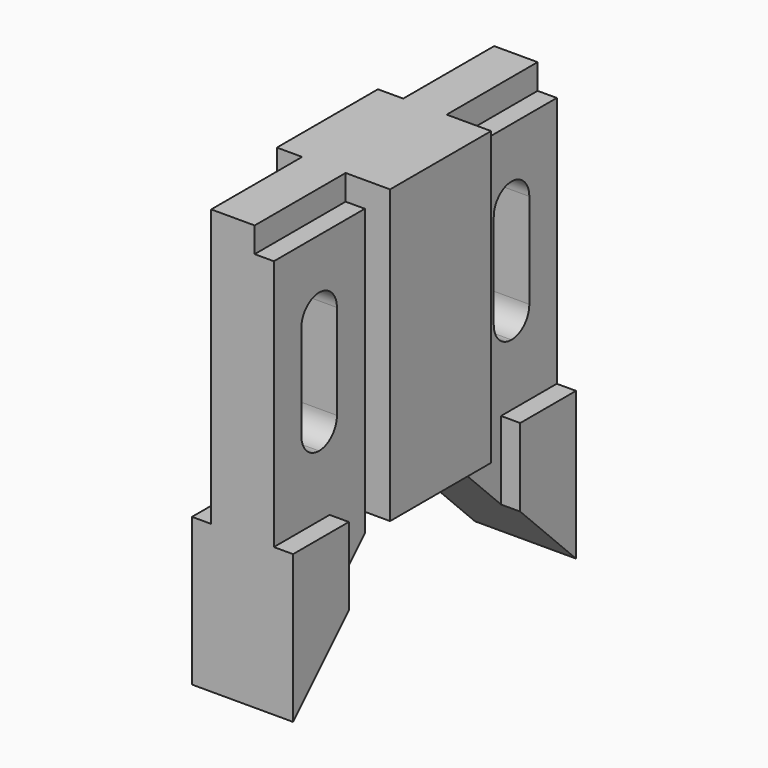
from build123d import *

# Parameters (mm, degrees)
F0_W      = 28.448
F0_H      = 73.406
F1_DEPTH  = 15.875
F2_W      = 28.575
F2_H      = 6.35
F3_DEPTH  = 7.874
F5_W      = 28.575
F5_H      = 6.35
F6_DEPTH  = 4.826
F8_DEPTH  = 12.7
F12_DEPTH = 40.132


with BuildPart() as f1:
    # F0 (on Front) → F1 (new body, symmetric)
    with BuildSketch(Plane.XZ):
        Rectangle(F0_W, F0_H)
    extrude(amount=F1_DEPTH, both=True)

    # F2 (on Right) → F3 (join, symmetric)
    with BuildSketch(Plane.YZ):
        Polygon((-15.875, -36.703), (-15.875, 30.353), (-44.45, 30.353), (-44.45, -32.893), (-26.924, -32.893), (-26.924, -52.4899314183), (-15.875, -41.4409314183), align=None)
        with Locations((-30.1625, 33.528)):
            Rectangle(F2_W, F2_H)
    extrude(amount=F3_DEPTH, both=True)

    # F5 (on offset) → F6 (cut)
    with BuildSketch(Plane.YZ.offset(7.874)):
        with Locations((-30.1625, 33.528)):
            Rectangle(F5_W, F5_H)
    extrude(amount=-F6_DEPTH, mode=Mode.SUBTRACT)

    # F7 (on Right) → F8 (join, symmetric)
    with BuildSketch(Plane.YZ):
        Polygon((-26.924, -32.893), (-44.45, -32.893), (-44.45, -70.0159314183), (-26.924, -52.4899314183), align=None)
    extrude(amount=F8_DEPTH, both=True)

    # F10: F1 across plane


with BuildPart() as f1_1:
    add(f1.part)
    add(f1.part.mirror(Plane.XZ))

    # F11 (on offset) → F12 (cut)
    with BuildSketch(Plane.YZ.offset(7.874)):
        with BuildLine():
            ThreePointArc((-30.226, 17.653), (-34.1773126933, 16.0163126933), (-35.814, 12.065))
            Line((-35.814, 12.065), (-35.814, -11.811))
            ThreePointArc((-35.814, -11.811), (-34.1773126933, -15.7623126933), (-30.226, -17.399))
            ThreePointArc((-30.226, -17.399), (-26.2746873067, -15.7623126933), (-24.638, -11.811))
            Line((-24.638, -11.811), (-24.638, 12.065))
            ThreePointArc((-24.638, 12.065), (-26.2746873067, 16.0163126933), (-30.226, 17.653))
        make_face()
        with BuildLine():
            ThreePointArc((30.226, -17.399), (34.1773126933, -15.7623126933), (35.814, -11.811))
            Line((35.814, -11.811), (35.814, 12.065))
            ThreePointArc((35.814, 12.065), (34.1773126933, 16.0163126933), (30.226, 17.653))
            ThreePointArc((30.226, 17.653), (26.2746873067, 16.0163126933), (24.638, 12.065))
            Line((24.638, 12.065), (24.638, -11.811))
            ThreePointArc((24.638, -11.811), (26.2746873067, -15.7623126933), (30.226, -17.399))
        make_face()
    extrude(amount=-F12_DEPTH, mode=Mode.SUBTRACT)


solid = f1_1.part
